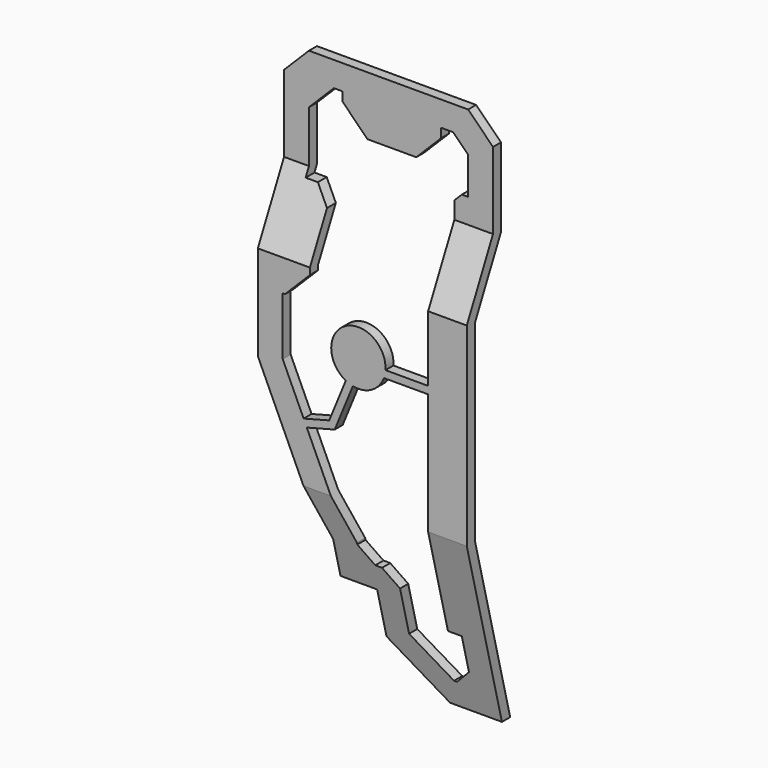
from build123d import *

# Parameters (mm, degrees)
F1_DEPTH = 25.4
F3_DEPTH = 30
F4_DEPTH = 30
F7_DEPTH = 25
F9_DEPTH = 40
F11_SIZE = 5
F12_SIZE = 3
F13_SIZE = 1.5


# Not quite as in the source:
# - a feature of the source that left no trace in its solid (it failed there, or was rolled back) is left out


with BuildPart() as f1:
    # F0 (on Front) → F1 (new body)
    with BuildSketch(Plane.XZ):
        Polygon((10.4166865349, 52.9566034675), (-31.557098031, 52.9566034675), (-31.557098031, 0), (-18.2580947876, -28.9524644613), (-18.2580947876, -36.2323522568), (-10.9038203955, -36.2323522568), (-10.9038203955, -45.4944968224), (0, -54.6278357506), (10.4166865349, -54.6278357506), align=None)
    extrude(amount=F1_DEPTH)


with BuildPart() as f3:
    # F2 (on Front) → F3 (new body, symmetric)
    with BuildSketch(Plane.XZ):
        with BuildLine():
            Line((-19.7998397052, 47.9566034675), (-26.557098031, 47.9566034675))
            Line((-26.557098031, 47.9566034675), (-26.557098031, 30.8428518474))
            Line((-26.557098031, 30.8428518474), (-21.0963413119, 30.8428518474))
            Line((-21.0963413119, 30.8428518474), (-21.0963413119, 12.7346292138))
            Line((-21.0963413119, 12.7346292138), (-26.557098031, 12.7346292138))
            Line((-26.557098031, 12.7346292138), (-26.557098031, 1.0934300149))
            Line((-26.557098031, 1.0934300149), (-22.3559527725, -8.0526320297))
            Line((-22.3559527725, -8.0526320297), (-17.2149640966, -6.7084824335))
            Line((-17.2149640966, -6.7084824335), (-13.8887305603, 1.4067513807))
            ThreePointArc((-13.8887305603, 1.4067513807), (-14.1854089296, 10.908286), (-5.9038203955, 6.2411166728))
            ThreePointArc((-5.9038203955, 6.2411166728), (-5.9071677422, 6.0500291804), (-5.9172056749, 5.8591761626))
            Line((-5.9172056749, 5.8591761626), (2.6482306421, 5.8591761626))
            Line((2.6482306421, 5.8591761626), (2.6482306421, 37.4990403652))
            Line((2.6482306421, 37.4990403652), (5.4166865349, 37.4990403652))
            Line((5.4166865349, 37.4990403652), (5.4166865349, 47.9566034675))
            Line((5.4166865349, 47.9566034675), (0, 47.9566034675))
            Line((0, 47.9566034675), (0, 41.127063334))
            Line((0, 41.127063334), (-19.7998397052, 41.127063334))
            Line((-19.7998397052, 41.127063334), (-19.7998397052, 47.9566034675))
        make_face()
    extrude(amount=F3_DEPTH, both=True)


with BuildPart() as f4:
    # F2 (on Front) → F4 (new body, symmetric)
    with BuildSketch(Plane.XZ):
        with BuildLine():
            Line((-16.1110319639, -7.9702737021), (-21.7201422185, -9.4368171549))
            Line((-21.7201422185, -9.4368171549), (-13.2580947876, -27.8590344464))
            Line((-13.2580947876, -27.8590344464), (-13.2580947876, -31.2323522568))
            Line((-13.2580947876, -31.2323522568), (-5.9038203955, -31.2323522568))
            Line((-5.9038203955, -31.2323522568), (-5.9038203955, -43.1603266307))
            Line((-5.9038203955, -43.1603266307), (1.8174038362, -49.6278357506))
            Line((1.8174038362, -49.6278357506), (5.4166865349, -49.6278357506))
            Line((5.4166865349, -49.6278357506), (5.4166865349, -39.5213142037))
            Line((5.4166865349, -39.5213142037), (2.6482306421, -39.5213142037))
            Line((2.6482306421, -39.5213142037), (2.6482306421, 4.3591761626))
            Line((2.6482306421, 4.3591761626), (-6.238670659, 4.3591761626))
            ThreePointArc((-6.238670659, 4.3591761626), (-8.7135994884, 1.4698551421), (-12.4751443179, 0.900443897))
            Line((-12.4751443179, 0.900443897), (-16.1110319639, -7.9702737021))
        make_face()
    extrude(amount=F4_DEPTH, both=True)


with BuildPart() as f1_1:
    add(f1.part)

    # F5: cut F3
    add(f3.part, mode=Mode.SUBTRACT)

    # F6: cut F4
    add(f4.part, mode=Mode.SUBTRACT)

    # F7 (add): a face of the model
    f7_faces = [f1_1.faces().sort_by_distance(p)[0] for p in [
        (-7.5880887423, 0, 6.6814576026),
    ]]
    extrude(f7_faces, amount=F7_DEPTH)


with BuildPart() as f9:
    # F8 (on Right) → F9 (new body, symmetric)
    with BuildSketch(Plane.YZ):
        Polygon((-5.4386107326, 32.0926371886), (-5.4386107326, 63.2104203105), (-7.4386107326, 63.2104203105), (-7.4386107326, 32.5547352223), (-14.0266608968, 19.0589928517), (-14.0266608968, -19.9610399589), (-3.9184388004, -59.6407970668), (-1.9803369667, -59.1470751993), (-12.0266608968, -19.7102989226), (-12.0266608968, 18.596894818), align=None)
    extrude(amount=F9_DEPTH, both=True)


with BuildPart() as f1_2:
    add(f1_1.part)

    # F10: intersect F9
    add(f9.part, mode=Mode.INTERSECT)

    # F11
    f11_edges = [f1_2.edges().sort_by_distance(p)[0] for p in [
        (-26.557098, -6.438611, 47.956603),
        (10.416687, -6.438611, 52.956603),
        (-31.557098, -6.438611, 52.956603),
        (0, -6.438611, 41.127063),
        (-19.79984, -6.438611, 41.127063),
        (-21.096341, -13.026661, 12.734629),
    ]]
    chamfer(f11_edges, length=F11_SIZE)

    # F12
    f12_edges = [f1_2.edges().sort_by_distance(p)[0] for p in [
        (5.416687, -6.438611, 47.956603),
        (-21.096341, -7.161491, 30.842852),
        (5.416687, -5.437254, -49.627836),
        (-5.90382, -10.123412, -31.232352),
        (-13.258095, -10.123412, -31.232352),
    ]]
    chamfer(f12_edges, length=F12_SIZE)

    # F13
    f13_edges = [f1_2.edges().sort_by_distance(p)[0] for p in [
        (2.648231, -6.438611, 37.49904),
    ]]
    chamfer(f13_edges, length=F13_SIZE)


solid = f1_2.part
